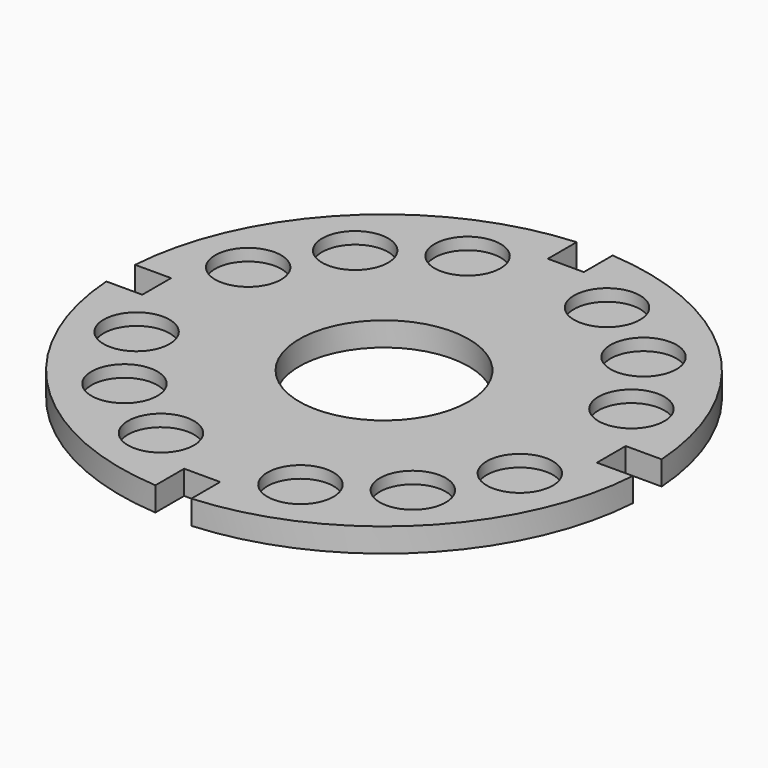
from build123d import *

# Parameters (mm, degrees)
F0_R            = 44.8437
F0_R_2          = 17.4625
F0_W            = 19.05
F0_H            = 6.35
F1_DEPTH        = 12.7
F2_DEPTH        = 6.35
F2_COPIES_COUNT = 4
F3_DEPTH        = 12.701
F3_COPIES_COUNT = 4
F5_DEPTH        = 25.4


# Not quite as in the source:
# - a pattern or mirror of a feature is missing from the dataset's text; its kind, count and spacing are read off the source's solid


with BuildPart() as f1:
    # F0 (on Top) → F1 (new body)
    with BuildSketch(Plane.XY):
        with BuildLine():
            ThreePointArc((-9.525, 139.3749058296), (-95.3557746023, -102.0948884617), (139.7, 0))
            ThreePointArc((139.7, 0), (102.0948884617, 95.3557746023), (9.525, 139.3749058296))
            Line((9.525, 139.3749058296), (9.525, 120.3249058296))
            Line((9.525, 120.3249058296), (9.525, 113.9749058296))
            Line((9.525, 113.9749058296), (-9.525, 113.9749058296))
            Line((-9.525, 113.9749058296), (-9.525, 120.3249058296))
            Line((-9.525, 120.3249058296), (-9.525, 139.3749058296))
        make_face()
        Circle(F0_R, mode=Mode.SUBTRACT)
        with Locations((101.4398184138, 36.921074472)):
            Circle(F0_R_2, mode=Mode.SUBTRACT)
        with Locations((36.921074472, 101.4398184138)):
            Circle(F0_R_2, mode=Mode.SUBTRACT)
        with Locations((76.3321770291, 76.3321770291)):
            Circle(F0_R_2, mode=Mode.SUBTRACT)
        with BuildLine():
            Line((9.525, 120.3249058296), (9.525, 139.3749058296))
            ThreePointArc((9.525, 139.3749058296), (0, 139.7), (-9.525, 139.3749058296))
            Line((-9.525, 139.3749058296), (-9.525, 120.3249058296))
            Line((-9.525, 120.3249058296), (9.525, 120.3249058296))
        make_face()
        with Locations((36.921074472, 101.4398184138)):
            Circle(F0_R_2)
        with Locations((76.3321770291, 76.3321770291)):
            Circle(F0_R_2)
        with Locations((101.4398184138, 36.921074472)):
            Circle(F0_R_2)
        with Locations((0, 117.1499058296)):
            Rectangle(F0_W, F0_H)
        Circle(F0_R)
    extrude(amount=-F1_DEPTH)

    # F0 (on Top) → F2 (cut)
    with BuildSketch(Plane.XY):
        with Locations((36.921074472, 101.4398184138)):
            Circle(F0_R_2)
        with Locations((76.3321770291, 76.3321770291)):
            Circle(F0_R_2)
        with Locations((101.4398184138, 36.921074472)):
            Circle(F0_R_2)
    f2 = extrude(amount=-F2_DEPTH, mode=Mode.SUBTRACT)

    # F2_copies: F2 ×4 about axis
    f2_copies_axis = Axis((0, 0, 0), (0, 0, 1))
    for i in range(1, F2_COPIES_COUNT):
        add(f2.rotate(f2_copies_axis, i * 360 / F2_COPIES_COUNT), mode=Mode.SUBTRACT)

    # F0 (on Top) → F3 (cut, through all)
    with BuildSketch(Plane.XY):
        with BuildLine():
            Line((9.525, 120.3249058296), (9.525, 139.3749058296))
            ThreePointArc((9.525, 139.3749058296), (0, 139.7), (-9.525, 139.3749058296))
            Line((-9.525, 139.3749058296), (-9.525, 120.3249058296))
            Line((-9.525, 120.3249058296), (9.525, 120.3249058296))
        make_face()
    f3 = extrude(amount=-F3_DEPTH, mode=Mode.SUBTRACT)

    # F3_copies: F3 ×4 about axis
    f3_copies_axis = Axis((0, 0, 0), (0, 0, 1))
    for i in range(1, F3_COPIES_COUNT):
        add(f3.rotate(f3_copies_axis, i * 360 / F3_COPIES_COUNT), mode=Mode.SUBTRACT)

    # F0 (on Top) → F5 (cut)
    with BuildSketch(Plane.XY):
        Circle(F0_R)
    extrude(amount=-F5_DEPTH, mode=Mode.SUBTRACT)


solid = f1.part
